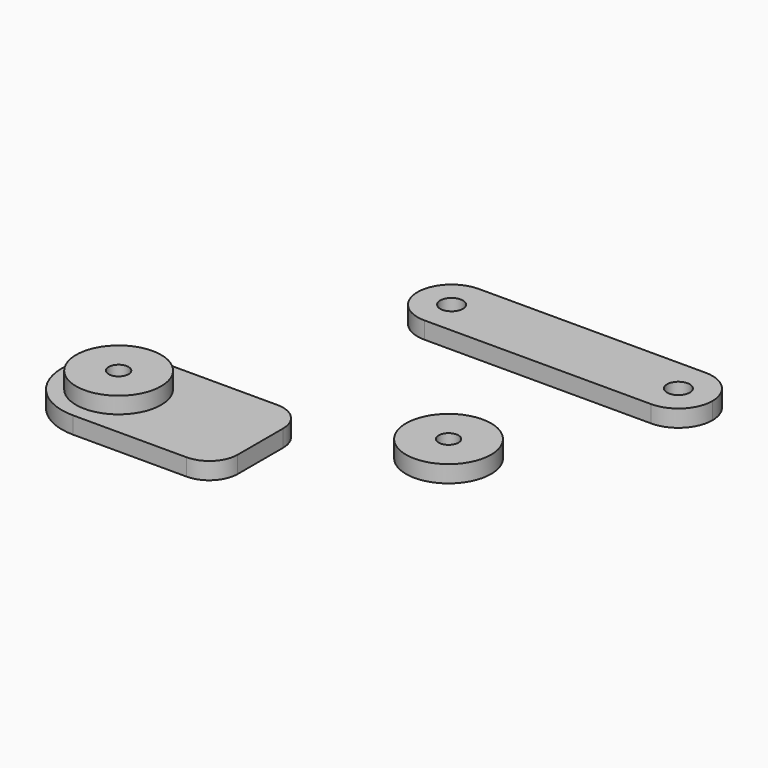
from build123d import *

# Parameters (mm, degrees)
F0_R     = 2
F1_DEPTH = 3
F3_DEPTH = 3
F4_R     = 7.5
F5_DEPTH = 2.9
F6_R     = 1.75
F7_DEPTH = 5.9
F8_R     = 7.5
F8_R_2   = 1.75
F9_DEPTH = 3
F10_R    = 5


with BuildPart() as f1:
    # F0 (on Top) → F1 (new body)
    with BuildSketch(Plane.XY):
        with BuildLine():
            ThreePointArc((0, -6), (4.2426406871, -4.2426406871), (6, 0))
            ThreePointArc((6, 0), (4.2426406871, 4.2426406871), (0, 6))
            ThreePointArc((0, 6), (-6, 0), (0, -6))
        make_face()
        Circle(F0_R, mode=Mode.SUBTRACT)
        with BuildLine():
            ThreePointArc((0, -6), (-6, 0), (0, 6))
            Line((0, 6), (-40, 6))
            ThreePointArc((-40, 6), (-35.7573593129, 4.2426406871), (-34, 0))
            ThreePointArc((-34, 0), (-35.7573593129, -4.2426406871), (-40, -6))
            Line((-40, -6), (0, -6))
        make_face()
        with BuildLine():
            ThreePointArc((-34, 0), (-35.7573593129, 4.2426406871), (-40, 6))
            ThreePointArc((-40, 6), (-46, 0), (-40, -6))
            ThreePointArc((-40, -6), (-35.7573593129, -4.2426406871), (-34, 0))
        make_face()
        with Locations((-40, 0)):
            Circle(F0_R, mode=Mode.SUBTRACT)
    extrude(amount=F1_DEPTH)


with BuildPart() as f3:
    # F2 (on Top) → F3 (new body)
    with BuildSketch(Plane.XY):
        with BuildLine():
            Line((-35.0382344763, -38.3426717669), (-60.0382344763, -38.3426717669))
            ThreePointArc((-60.0382344763, -38.3426717669), (-70.0382344763, -48.3426717669), (-60.0382344763, -58.3426717669))
            Line((-60.0382344763, -58.3426717669), (-35.0382344763, -58.3426717669))
            Line((-35.0382344763, -58.3426717669), (-35.0382344763, -38.3426717669))
        make_face()
    extrude(amount=F3_DEPTH)

    # F4 (on face) → F5 (join)
    with BuildSketch(Plane.XY.offset(3)):
        with Locations((-60.0382344763, -48.3426717669)):
            Circle(F4_R)
    extrude(amount=F5_DEPTH)

    # F6 (on face) → F7 (cut, through all)
    with BuildSketch(Plane.XY.offset(5.9)):
        with Locations((-60.0382344763, -48.3426717669)):
            Circle(F6_R)
    extrude(amount=-F7_DEPTH, mode=Mode.SUBTRACT)

    # F10
    f10_edges = [f3.edges().sort_by_distance(p)[0] for p in [
        (-35.038234, -38.342672, 1.5),
        (-35.038234, -58.342672, 1.5),
    ]]
    fillet(f10_edges, radius=F10_R)


with BuildPart() as f9:
    # F8 (on Top) → F9 (new body)
    with BuildSketch(Plane.XY):
        with Locations((-15.2930086479, -31.5495021641)):
            Circle(F8_R)
        with Locations((-15.2930086479, -31.5495021641)):
            Circle(F8_R_2, mode=Mode.SUBTRACT)
    extrude(amount=F9_DEPTH)


solid = Compound([f1.part, f3.part, f9.part])
